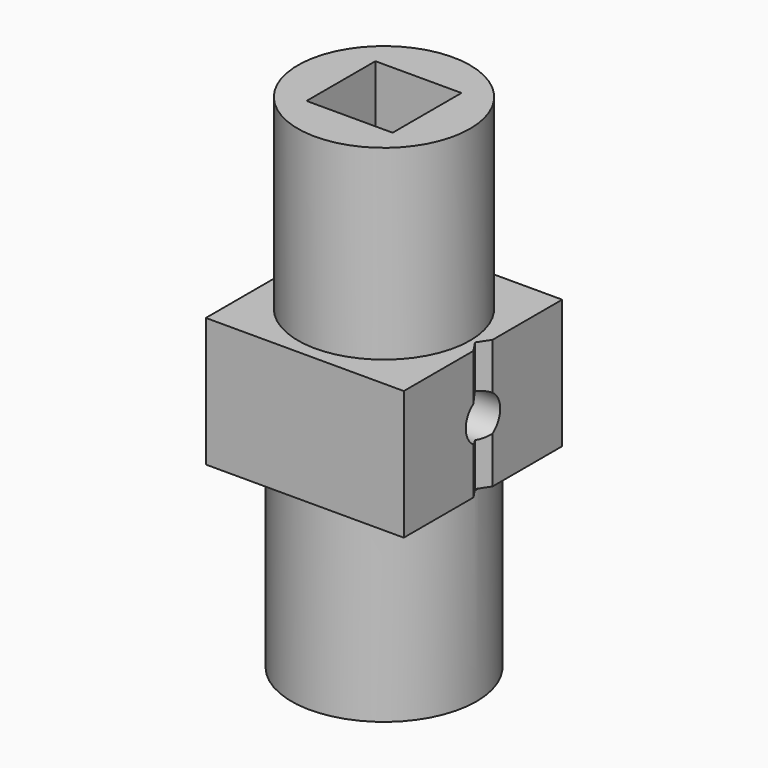
from build123d import *

# Parameters (mm, degrees)
F0_W      = 13.8
F0_H      = 13.8
F1_DEPTH  = 4.5
F2_R      = 6
F3_DEPTH  = 13
F4_R      = 6.45
F5_DEPTH  = 13
F6_R      = 1.5
F7_DEPTH  = 13.801
F9_DEPTH  = 22.001
F10_W     = 6
F10_H     = 6
F11_DEPTH = 6.5
F13_DEPTH = 6.5


with BuildPart() as f1:
    # F0 (on Top) → F1 (new body, symmetric)
    with BuildSketch(Plane.XY):
        Rectangle(F0_W, F0_H)
    extrude(amount=F1_DEPTH, both=True)

    # F2 (on face) → F3 (join)
    with BuildSketch(Plane.XY.offset(4.5)):
        Circle(F2_R)
    extrude(amount=F3_DEPTH)

    # F4 (on face) → F5 (join)
    with BuildSketch(Plane(origin=(0, 0, -4.5), x_dir=(1, 0, 0), z_dir=(0, 0, -1))):
        Circle(F4_R)
    extrude(amount=F5_DEPTH)

    # F6 (on face) → F7 (cut, through all)
    with BuildSketch(Plane.YZ.offset(6.9)):
        Circle(F6_R)
    extrude(amount=-F7_DEPTH, mode=Mode.SUBTRACT)

    # F8 (on face) → F9 (cut, through all)
    with BuildSketch(Plane(origin=(0, 0, -4.5), x_dir=(1, 0, 0), z_dir=(0, 0, -1))):
        Polygon((6.9, 0.8288529099), (6.3405334204, 0), (6.9, -0.8288529099), align=None)
        Polygon((-6.9, -0.7952927344), (-6.2937744095, 0), (-6.9, 0.7952927344), align=None)
    extrude(amount=-F9_DEPTH, mode=Mode.SUBTRACT)

    # F10 (on face) → F11 (cut)
    with BuildSketch(Plane.XY.offset(17.5)):
        Rectangle(F10_W, F10_H)
    extrude(amount=-F11_DEPTH, mode=Mode.SUBTRACT)

    # F12 (on face) → F13 (cut)
    with BuildSketch(Plane(origin=(0, 0, -17.5), x_dir=(1, 0, 0), z_dir=(0, 0, -1))):
        with BuildLine():
            ThreePointArc((3.5496478699, -2.15), (3.9970951114, -1.1161230533), (4.15, 0))
            ThreePointArc((4.15, 0), (-1.1161230533, 3.9970951114), (-3.5496478699, -2.15))
            Line((-3.5496478699, -2.15), (0, -2.15))
            Line((0, -2.15), (3.5496478699, -2.15))
        make_face()
    extrude(amount=-F13_DEPTH, mode=Mode.SUBTRACT)


solid = f1.part
